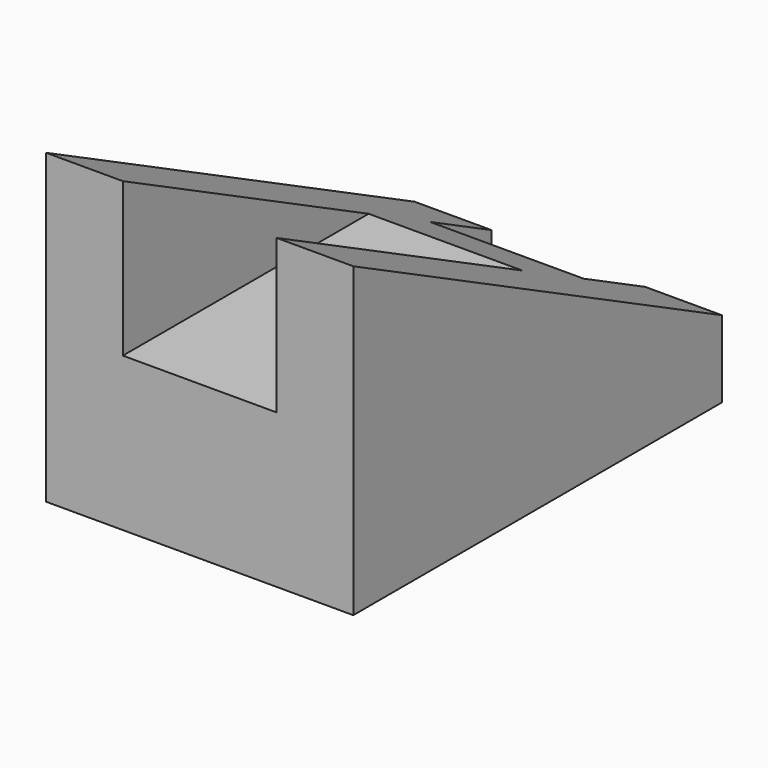
from build123d import *

# Parameters (mm, degrees)
F1_DEPTH      = 30
F3_DEPTH      = 10.001
F3_DEPTH_BACK = 10.001
F4_W          = 10
F4_H          = 5
F5_DEPTH      = 20.001


with BuildPart() as f1:
    # F0 (on Front) → F1 (new body)
    with BuildSketch(Plane.XZ):
        Polygon((-10, 0), (0, 0), (10, 0), (10, 20), (5, 20), (5, 10), (-5, 10), (-5, 20), (-10, 20), align=None)
    extrude(amount=-F1_DEPTH)

    # F2 (on Right) → F3 (cut, two sides)
    with BuildSketch(Plane.YZ) as f3_sk:
        Polygon((30, 5), (30, 20), (0, 20), align=None)
    extrude(amount=-F3_DEPTH, mode=Mode.SUBTRACT)
    extrude(f3_sk.sketch, amount=F3_DEPTH_BACK, mode=Mode.SUBTRACT)

    # F4 (on face) → F5 (cut, through all)
    with BuildSketch(Plane(origin=(0, 0, 0), x_dir=(1, 0, 0), z_dir=(0, 0, -1))):
        with Locations((0, -27.5)):
            Rectangle(F4_W, F4_H)
    extrude(amount=-F5_DEPTH, mode=Mode.SUBTRACT)


solid = f1.part
